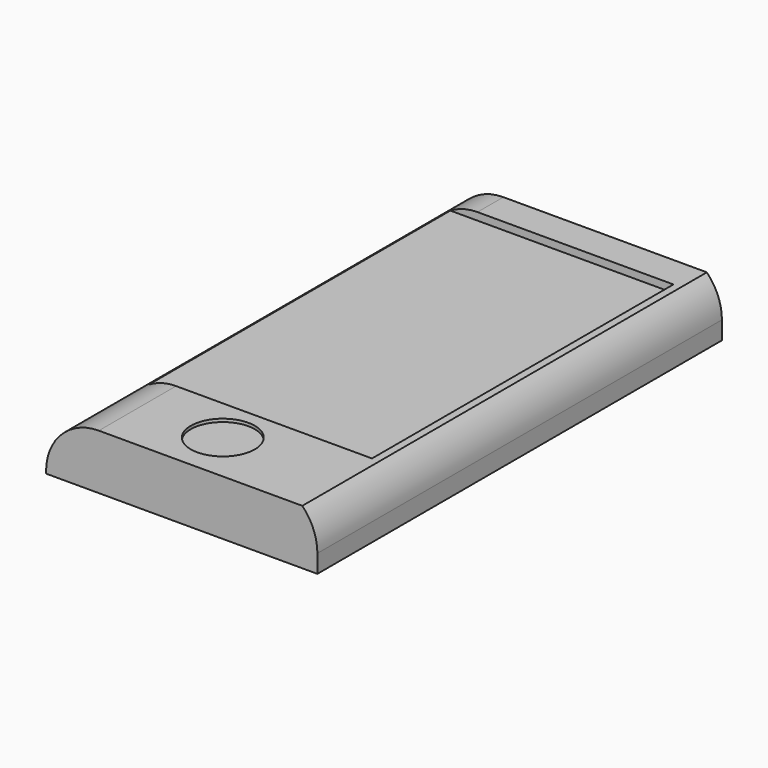
from build123d import *

# Parameters (mm, degrees)
F0_W        = 36
F0_H        = 67.1
F1_DEPTH    = 7.3
F2_R        = 4.2454518292
F3_DEPTH    = 0.4
F5_SIZE     = 2
F6_T1_DEPTH = 81.5974746831
F4_W        = 30
F4_H        = 50
F7_DEPTH    = 1
F8_T1_DEPTH = 102.1


# Not quite as in the source:
# - a fillet or chamfer that OpenCascade refuses, or shapes differently, is made with other operations: its cross-section is extruded or revolved along the edge and cut away or added


with BuildPart() as f1:
    # F0 (on Top) → F1 (new body)
    with BuildSketch(Plane.XY):
        Rectangle(F0_W, F0_H)
    extrude(amount=F1_DEPTH)

    # F2 (on face) → F3 (cut)
    with BuildSketch(Plane.XY.offset(7.3)):
        with Locations((0, -26.7354752868)):
            Circle(F2_R)
    extrude(amount=-F3_DEPTH, mode=Mode.SUBTRACT)

    # F5
    f5_edges = [f1.edges().sort_by_distance(p)[0] for p in [
        (18, 0, 7.3),
    ]]
    chamfer(f5_edges, length=F5_SIZE)

    # F6: fillet of radius 7 on 1 edges, made by hand

    # F6_s2 → F6_t1 (cut)
    with BuildSketch(Plane.XZ.offset(-40.7987373415)):
        with BuildLine():
            ThreePointArc((18, 2.4005050634), (17.4671567276, 5.0792890899), (15.9497474683, 7.3502525317))
            Line((15.9497474683, 7.3502525317), (18, 5.3))
            Line((18, 5.3), (18, 2.4005050634))
        make_face()
    extrude(amount=F6_T1_DEPTH, mode=Mode.SUBTRACT)

    # F4 (on face) → F7 (cut)
    with BuildSketch(Plane.XY.offset(7.3)):
        with Locations((0, 4.2591368308)):
            Rectangle(F4_W, F4_H)
    extrude(amount=-F7_DEPTH, mode=Mode.SUBTRACT)

    # F8: fillet of radius 7 on 1 edges, made by hand

    # F8_s2 → F8_t1 (cut)
    with BuildSketch(Plane.XZ.offset(-51.05)):
        with BuildLine():
            ThreePointArc((-18, 0.3), (-15.9497474683, 5.2497474683), (-11, 7.3))
            Line((-11, 7.3), (-18, 7.3))
            Line((-18, 7.3), (-18, 0.3))
        make_face()
    extrude(amount=F8_T1_DEPTH, mode=Mode.SUBTRACT)


solid = f1.part
